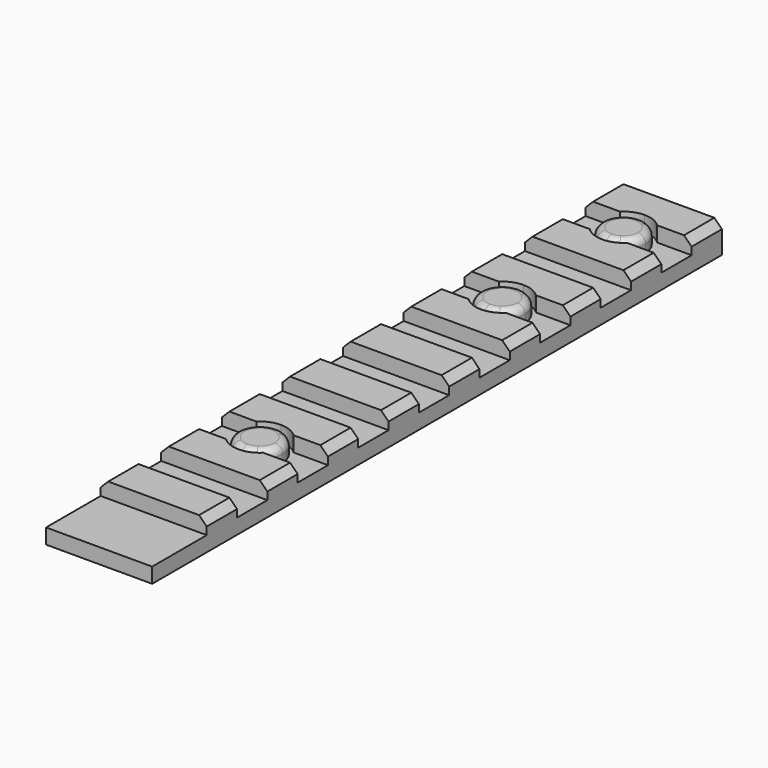
from build123d import *

# Parameters (mm, degrees)
F0_W     = 14
F0_H     = 94
F1_DEPTH = 2
F2_W     = 7
F2_H     = 5
F3_DEPTH = 2
F4_SIZE  = 1
F5_R     = 1


with BuildPart() as f1:
    # F0 (on Top) → F1 (new body)
    with BuildSketch(Plane.XY):
        with Locations((-7, 11.0699324605)):
            Rectangle(F0_W, F0_H)
    extrude(amount=F1_DEPTH)

    # F2 (on face) → F3 (join)
    with BuildSketch(Plane.XY.offset(2)):
        with BuildLine():
            Line((-7, 58.0699324605), (-14, 58.0699324605))
            Line((-14, 58.0699324605), (-14, 53.0699324605))
            Line((-14, 53.0699324605), (-9.4494897428, 53.0699324605))
            ThreePointArc((-9.4494897428, 53.0699324605), (-8.3228756555, 53.8103028097), (-7, 54.0699324605))
            Line((-7, 54.0699324605), (-7, 58.0699324605))
        make_face()
        with BuildLine():
            Line((0, 58.0699324605), (-7, 58.0699324605))
            Line((-7, 58.0699324605), (-7, 54.0699324605))
            ThreePointArc((-7, 54.0699324605), (-5.6771243445, 53.8103028097), (-4.5505102572, 53.0699324605))
            Line((-4.5505102572, 53.0699324605), (0, 53.0699324605))
            Line((0, 53.0699324605), (0, 58.0699324605))
        make_face()
        with BuildLine():
            Line((-9.4494897428, 48.0699324605), (-14, 48.0699324605))
            Line((-14, 48.0699324605), (-14, 43.0699324605))
            Line((-14, 43.0699324605), (-7, 43.0699324605))
            Line((-7, 43.0699324605), (-7, 47.0699324605))
            ThreePointArc((-7, 47.0699324605), (-8.3228756555, 47.3295621113), (-9.4494897428, 48.0699324605))
        make_face()
        with BuildLine():
            ThreePointArc((-4.5505102572, 48.0699324605), (-5.6771243445, 47.3295621113), (-7, 47.0699324605))
            Line((-7, 47.0699324605), (-7, 43.0699324605))
            Line((-7, 43.0699324605), (0, 43.0699324605))
            Line((0, 43.0699324605), (0, 48.0699324605))
            Line((0, 48.0699324605), (-4.5505102572, 48.0699324605))
        make_face()
        with BuildLine():
            Line((0, 38.0699324605), (-7, 38.0699324605))
            Line((-7, 38.0699324605), (-7, 34.0699324605))
            ThreePointArc((-7, 34.0699324605), (-5.6771243445, 33.8103028097), (-4.5505102572, 33.0699324605))
            Line((-4.5505102572, 33.0699324605), (0, 33.0699324605))
            Line((0, 33.0699324605), (0, 38.0699324605))
        make_face()
        with BuildLine():
            Line((-7, 38.0699324605), (-14, 38.0699324605))
            Line((-14, 38.0699324605), (-14, 33.0699324605))
            Line((-14, 33.0699324605), (-9.4494897428, 33.0699324605))
            ThreePointArc((-9.4494897428, 33.0699324605), (-8.3228756555, 33.8103028097), (-7, 34.0699324605))
            Line((-7, 34.0699324605), (-7, 38.0699324605))
        make_face()
        with BuildLine():
            Line((-9.4494897428, 28.0699324605), (-14, 28.0699324605))
            Line((-14, 28.0699324605), (-14, 23.0699324605))
            Line((-14, 23.0699324605), (-7, 23.0699324605))
            Line((-7, 23.0699324605), (-7, 27.0699324605))
            ThreePointArc((-7, 27.0699324605), (-8.3228756555, 27.3295621113), (-9.4494897428, 28.0699324605))
        make_face()
        with BuildLine():
            Line((0, 23.0699324605), (0, 28.0699324605))
            Line((0, 28.0699324605), (-4.5505102572, 28.0699324605))
            ThreePointArc((-4.5505102572, 28.0699324605), (-5.6771243445, 27.3295621113), (-7, 27.0699324605))
            Line((-7, 27.0699324605), (-7, 23.0699324605))
            Line((-7, 23.0699324605), (0, 23.0699324605))
        make_face()
        with Locations((-10.5, 15.5699324605)):
            Rectangle(F2_W, F2_H)
        with Locations((-3.5, 15.5699324605)):
            Rectangle(F2_W, F2_H)
        with Locations((-10.5, 5.5699324605)):
            Rectangle(F2_W, F2_H)
        with Locations((-3.5, 5.5699324605)):
            Rectangle(F2_W, F2_H)
        with BuildLine():
            Line((-7, -1.9300675395), (-14, -1.9300675395))
            Line((-14, -1.9300675395), (-14, -6.9300675395))
            Line((-14, -6.9300675395), (-9.4494897428, -6.9300675395))
            ThreePointArc((-9.4494897428, -6.9300675395), (-8.3228756555, -6.1896971903), (-7, -5.9300675395))
            Line((-7, -5.9300675395), (-7, -1.9300675395))
        make_face()
        with BuildLine():
            Line((0, -1.9300675395), (-7, -1.9300675395))
            Line((-7, -1.9300675395), (-7, -5.9300675395))
            ThreePointArc((-7, -5.9300675395), (-5.6771243445, -6.1896971903), (-4.5505102572, -6.9300675395))
            Line((-4.5505102572, -6.9300675395), (0, -6.9300675395))
            Line((0, -6.9300675395), (0, -1.9300675395))
        make_face()
        with BuildLine():
            Line((-9.4494897428, -11.9300675395), (-14, -11.9300675395))
            Line((-14, -11.9300675395), (-14, -16.9300675395))
            Line((-14, -16.9300675395), (-7, -16.9300675395))
            Line((-7, -16.9300675395), (-7, -12.9300675395))
            ThreePointArc((-7, -12.9300675395), (-8.3228756555, -12.6704378887), (-9.4494897428, -11.9300675395))
        make_face()
        with BuildLine():
            Line((0, -16.9300675395), (0, -11.9300675395))
            Line((0, -11.9300675395), (-4.5505102572, -11.9300675395))
            ThreePointArc((-4.5505102572, -11.9300675395), (-5.6771243445, -12.6704378887), (-7, -12.9300675395))
            Line((-7, -12.9300675395), (-7, -16.9300675395))
            Line((-7, -16.9300675395), (0, -16.9300675395))
        make_face()
        with Locations((-10.5, -24.4300675395)):
            Rectangle(F2_W, F2_H)
        with Locations((-3.5, -24.4300675395)):
            Rectangle(F2_W, F2_H)
        with BuildLine():
            Line((-7, 53.0699324605), (-8.5114243945, 53.0699324605))
            ThreePointArc((-8.5114243945, 53.0699324605), (-9.9213701751, 50.5699324605), (-8.5114243945, 48.0699324605))
            Line((-8.5114243945, 48.0699324605), (-7, 48.0699324605))
            Line((-7, 48.0699324605), (-7, 53.0699324605))
        make_face()
        with BuildLine():
            Line((-5.4885756055, 53.0699324605), (-7, 53.0699324605))
            Line((-7, 53.0699324605), (-7, 48.0699324605))
            Line((-7, 48.0699324605), (-5.4885756055, 48.0699324605))
            ThreePointArc((-5.4885756055, 48.0699324605), (-4.455414194, 49.1348412522), (-4.0786298249, 50.5699324605))
            ThreePointArc((-4.0786298249, 50.5699324605), (-4.455414194, 52.0050236688), (-5.4885756055, 53.0699324605))
        make_face()
        with BuildLine():
            ThreePointArc((-5.4885756055, 53.0699324605), (-6.2154688463, 53.3839890642), (-7, 53.4913026356))
            Line((-7, 53.4913026356), (-7, 53.0699324605))
            Line((-7, 53.0699324605), (-5.4885756055, 53.0699324605))
        make_face()
        with BuildLine():
            ThreePointArc((-7, 53.4913026356), (-7.7845311537, 53.3839890642), (-8.5114243945, 53.0699324605))
            Line((-8.5114243945, 53.0699324605), (-7, 53.0699324605))
            Line((-7, 53.0699324605), (-7, 53.4913026356))
        make_face()
        with BuildLine():
            Line((-7, 48.0699324605), (-8.5114243945, 48.0699324605))
            ThreePointArc((-8.5114243945, 48.0699324605), (-7.7845311537, 47.7558758567), (-7, 47.6485622853))
            Line((-7, 47.6485622853), (-7, 48.0699324605))
        make_face()
        with BuildLine():
            Line((-5.4885756055, 48.0699324605), (-7, 48.0699324605))
            Line((-7, 48.0699324605), (-7, 47.6485622853))
            ThreePointArc((-7, 47.6485622853), (-6.2154688463, 47.7558758567), (-5.4885756055, 48.0699324605))
        make_face()
        with BuildLine():
            Line((-7, 33.0699324605), (-7, 33.5699324605))
            ThreePointArc((-7, 33.5699324605), (-7.8660254038, 33.4422137837), (-8.6583123952, 33.0699324605))
            Line((-8.6583123952, 33.0699324605), (-7, 33.0699324605))
        make_face()
        with BuildLine():
            ThreePointArc((-5.3416876048, 33.0699324605), (-6.1339745962, 33.4422137837), (-7, 33.5699324605))
            Line((-7, 33.5699324605), (-7, 33.0699324605))
            Line((-7, 33.0699324605), (-5.3416876048, 33.0699324605))
        make_face()
        with BuildLine():
            Line((-5.3416876048, 33.0699324605), (-7, 33.0699324605))
            Line((-7, 33.0699324605), (-7, 28.0699324605))
            Line((-7, 28.0699324605), (-5.3416876048, 28.0699324605))
            ThreePointArc((-5.3416876048, 28.0699324605), (-4.3566179631, 29.151295295), (-4, 30.5699324605))
            ThreePointArc((-4, 30.5699324605), (-4.3566179631, 31.9885696259), (-5.3416876048, 33.0699324605))
        make_face()
        with BuildLine():
            Line((-7, 33.0699324605), (-8.6583123952, 33.0699324605))
            ThreePointArc((-8.6583123952, 33.0699324605), (-10, 30.5699324605), (-8.6583123952, 28.0699324605))
            Line((-8.6583123952, 28.0699324605), (-7, 28.0699324605))
            Line((-7, 28.0699324605), (-7, 33.0699324605))
        make_face()
        with BuildLine():
            Line((-7, 28.0699324605), (-8.6583123952, 28.0699324605))
            ThreePointArc((-8.6583123952, 28.0699324605), (-7.8660254038, 27.6976511372), (-7, 27.5699324605))
            Line((-7, 27.5699324605), (-7, 28.0699324605))
        make_face()
        with BuildLine():
            Line((-5.3416876048, 28.0699324605), (-7, 28.0699324605))
            Line((-7, 28.0699324605), (-7, 27.5699324605))
            ThreePointArc((-7, 27.5699324605), (-6.1339745962, 27.6976511372), (-5.3416876048, 28.0699324605))
        make_face()
        with BuildLine():
            Line((-7, -6.9300675395), (-7, -6.4300675395))
            ThreePointArc((-7, -6.4300675395), (-7.8660254038, -6.5577862163), (-8.6583123952, -6.9300675395))
            Line((-8.6583123952, -6.9300675395), (-7, -6.9300675395))
        make_face()
        with BuildLine():
            ThreePointArc((-5.3416876048, -6.9300675395), (-6.1339745962, -6.5577862163), (-7, -6.4300675395))
            Line((-7, -6.4300675395), (-7, -6.9300675395))
            Line((-7, -6.9300675395), (-5.3416876048, -6.9300675395))
        make_face()
        with BuildLine():
            Line((-5.3416876048, -6.9300675395), (-7, -6.9300675395))
            Line((-7, -6.9300675395), (-7, -11.9300675395))
            Line((-7, -11.9300675395), (-5.3416876048, -11.9300675395))
            ThreePointArc((-5.3416876048, -11.9300675395), (-4.3566179631, -10.848704705), (-4, -9.4300675395))
            ThreePointArc((-4, -9.4300675395), (-4.3566179631, -8.0114303741), (-5.3416876048, -6.9300675395))
        make_face()
        with BuildLine():
            Line((-7, -6.9300675395), (-8.6583123952, -6.9300675395))
            ThreePointArc((-8.6583123952, -6.9300675395), (-10, -9.4300675395), (-8.6583123952, -11.9300675395))
            Line((-8.6583123952, -11.9300675395), (-7, -11.9300675395))
            Line((-7, -11.9300675395), (-7, -6.9300675395))
        make_face()
        with BuildLine():
            Line((-7, -11.9300675395), (-8.6583123952, -11.9300675395))
            ThreePointArc((-8.6583123952, -11.9300675395), (-7.8660254038, -12.3023488628), (-7, -12.4300675395))
            Line((-7, -12.4300675395), (-7, -11.9300675395))
        make_face()
        with BuildLine():
            Line((-5.3416876048, -11.9300675395), (-7, -11.9300675395))
            Line((-7, -11.9300675395), (-7, -12.4300675395))
            ThreePointArc((-7, -12.4300675395), (-6.1339745962, -12.3023488628), (-5.3416876048, -11.9300675395))
        make_face()
    extrude(amount=F3_DEPTH)

    # F4
    f4_edges = [f1.edges().sort_by_distance(p)[0] for p in [
        (-14, 55.569932, 4),
        (-14, 45.569932, 4),
        (-14, 35.569932, 4),
        (-14, 25.569932, 4),
        (-14, 15.569932, 4),
        (-14, 5.569932, 4),
        (-14, -4.430068, 4),
        (-14, -14.430068, 4),
        (-14, -24.430068, 4),
        (0, -24.430068, 4),
        (0, -14.430068, 4),
        (0, -4.430068, 4),
        (0, 5.569932, 4),
        (0, 15.569932, 4),
        (0, 25.569932, 4),
        (0, 35.569932, 4),
        (0, 45.569932, 4),
        (0, 55.569932, 4),
    ]]
    chamfer(f4_edges, length=F4_SIZE)

    # F5
    f5_edges = [f1.edges().sort_by_distance(p)[0] for p in [
        (-5.341688, -11.930068, 4),
        (-5.341688, 28.069932, 4),
        (-5.488576, 53.069932, 4),
    ]]
    fillet(f5_edges, radius=F5_R)


solid = f1.part
